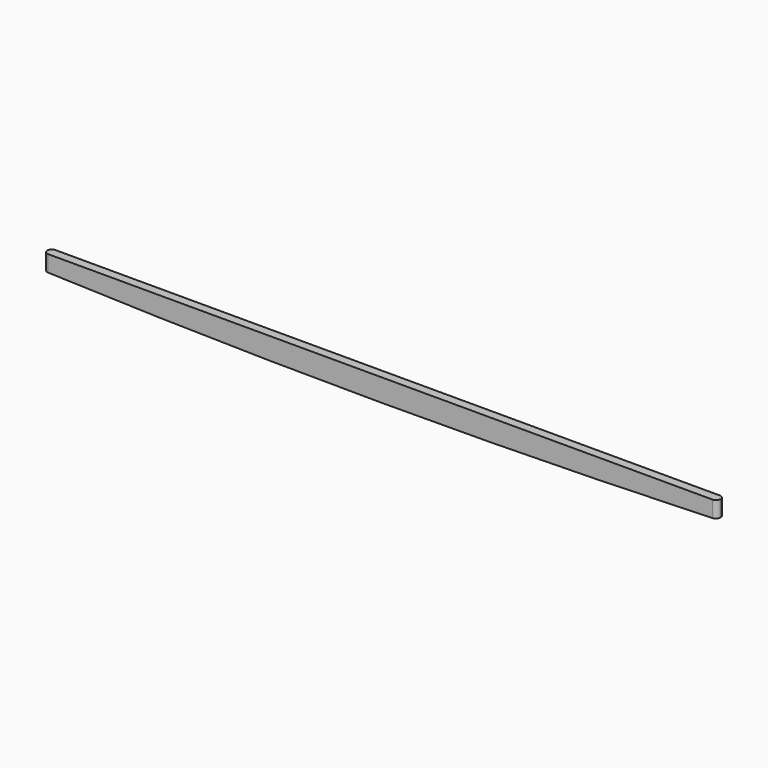
from build123d import *

# Parameters (mm, degrees)
F1_DEPTH = 2.54
F2_R     = 2.53999


# Not quite as in the source:
# - a fillet or chamfer is up to 0.001 mm smaller than in the source, because OpenCascade refuses the exact size


with BuildPart() as f1:
    # F0 (on Front) → F1 (new body, symmetric)
    with BuildSketch(Plane.XZ):
        with BuildLine():
            Line((-128.9416431369, 0), (-319.4416431369, 0))
            Line((-319.4416431369, 0), (-319.4416431369, -9.126868379))
            ThreePointArc((-319.4416431369, -9.126868379), (-224.2083966105, -11.8066385421), (-128.9416431369, -12.7))
            Line((-128.9416431369, -12.7), (-128.9416431369, 0))
        make_face()
        with BuildLine():
            Line((61.5583568631, 0), (-128.9416431369, 0))
            Line((-128.9416431369, 0), (-128.9416431369, -12.7))
            ThreePointArc((-128.9416431369, -12.7), (-33.6748896633, -11.8066385421), (61.5583568631, -9.126868379))
            Line((61.5583568631, -9.126868379), (61.5583568631, 0))
        make_face()
    extrude(amount=F1_DEPTH, both=True)

    # F2 (radius 2.54 in the source; OpenCascade refuses exactly that, so slightly less here)
    f2_edges = [f1.edges().sort_by_distance(p)[0] for p in [
        (-319.441643, -2.54, -4.563434),
        (-319.441643, 2.54, -4.563434),
        (61.558357, -2.54, -4.563434),
        (61.558357, 2.54, -4.563434),
    ]]
    fillet(f2_edges, radius=F2_R)


solid = f1.part
